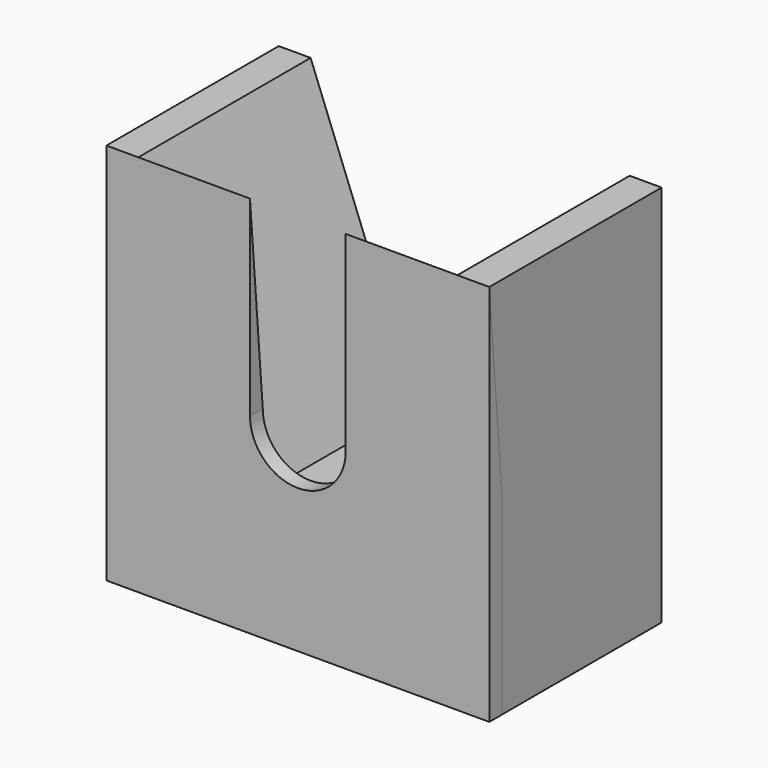
from build123d import *

# Parameters (mm, degrees)
F1_DEPTH = 3375
F2_W     = 2250
F2_H     = 3000
F3_DEPTH = 250
F4_SIZE2 = 249.99999
F4_SIZE  = 2999.99999
F5_SIZE2 = 249.99999
F5_SIZE  = 2999.99999
F6_DEPTH = 250


# Not quite as in the source:
# - a fillet or chamfer is up to 0.001 mm smaller than in the source, because OpenCascade refuses the exact size


with BuildPart() as f1:
    # F0 (on Front) → F1 (new body)
    with BuildSketch(Plane.XZ):
        Polygon((3000, -3000), (3000, 3000), (2500, 3000), (856.9015333837, -1250), (-856.9015333837, -1250), (-2500, 3000), (-3000, 3000), (-3000, -3000), align=None)
    extrude(amount=-F1_DEPTH)


with BuildPart() as f3:
    # F2 (on Front) → F3 (new body)
    with BuildSketch(Plane.XZ):
        with Locations((1875, 1500)):
            Rectangle(F2_W, F2_H)
    extrude(amount=-F3_DEPTH)

    # F4 (size 3000 and 250 in the source; OpenCascade refuses exactly that, so slightly less here)
    f4_edges = [f3.edges().sort_by_distance(p)[0] for p in [
        (1875, 250, 3000),
    ]]
    f4_side = f3.faces().sort_by_distance((1875, 250, 1500))[0]
    chamfer(f4_edges, length=F4_SIZE, length2=F4_SIZE2, reference=f4_side)



with BuildPart() as f3b:
    # F2 (on Front) → F3, piece 2 (new body)
    with BuildSketch(Plane.XZ):
        with Locations((-1875, 1500)):
            Rectangle(F2_W, F2_H)
    extrude(amount=-F3_DEPTH)

    # F5 (size 3000 and 250 in the source; OpenCascade refuses exactly that, so slightly less here)
    f5_edges = [f3b.edges().sort_by_distance(p)[0] for p in [
        (-1875, 250, 3000),
    ]]
    f5_side = f3b.faces().sort_by_distance((-1875, 250, 1500))[0]
    chamfer(f5_edges, length=F5_SIZE, length2=F5_SIZE2, reference=f5_side)


with BuildPart() as f3_1:
    add(f3.part)

    add(f3b.part)  # F6 merges F3b
    # F2 (on Front) → F6 (join)
    with BuildSketch(Plane.XZ):
        with BuildLine():
            Line((-3000, 0), (-3000, -3000))
            Line((-3000, -3000), (3000, -3000))
            Line((3000, -3000), (3000, 0))
            Line((3000, 0), (750, 0))
            ThreePointArc((750, 0), (0, -750), (-750, 0))
            Line((-750, 0), (-3000, 0))
        make_face()
    extrude(amount=-F6_DEPTH)


solid = Compound([f1.part, f3_1.part])
